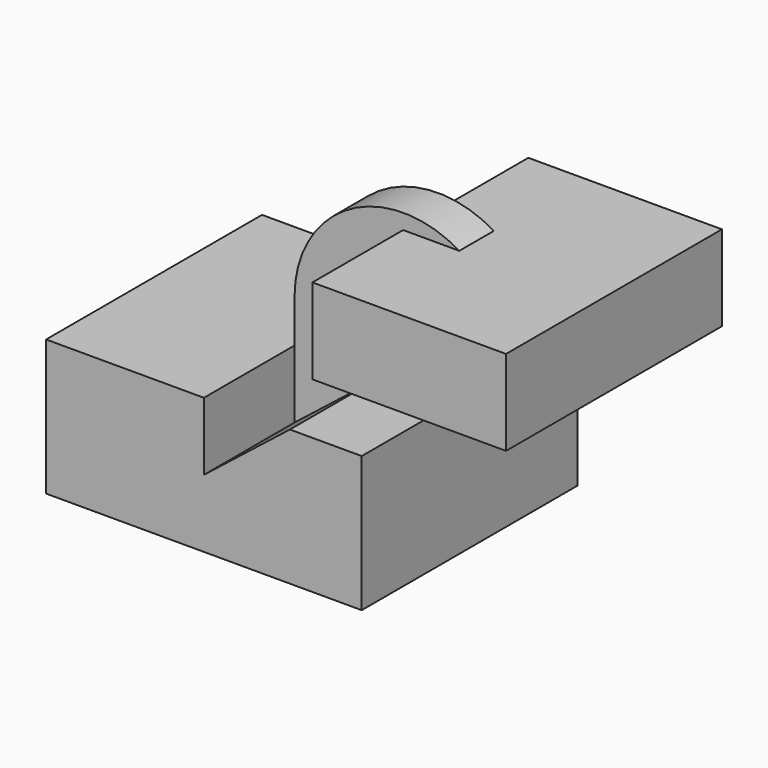
from build123d import *

# Parameters (mm, degrees)
F1_DEPTH = 62.5
F2_DEPTH = 10


with BuildPart() as f1:
    # F0 (on Front) → F1 (new body, symmetric)
    with BuildSketch(Plane.XZ):
        with BuildLine():
            Line((0, 31.4277224243), (-73.1017515063, 31.4277224243))
            Line((-73.1017515063, 31.4277224243), (-73.1017515063, -31.4277224243))
            Line((-73.1017515063, -31.4277224243), (73.1017515063, -31.4277224243))
            Line((73.1017515063, -31.4277224243), (73.1017515063, 31.4277224243))
            Line((73.1017515063, 31.4277224243), (39.8282436226, 31.4277224243))
            add(Edge.make_bspline(
                [(0, 0), (13.2760812075, 10.4759074748), (26.552162415, 20.9518149495), (39.8282436226, 31.4277224243)],
                knots=[0, 0, 0, 0, 50.7345121868, 50.7345121868, 50.7345121868, 50.7345121868], degree=3))
            Line((0, 0), (0, 31.4277224243))
        make_face()
    extrude(amount=F1_DEPTH, both=True)


with BuildPart() as f1b:
    # F0 (on Front) → F1, piece 2 (new body, symmetric)
    with BuildSketch(Plane.XZ):
        with BuildLine():
            add(Edge.make_bspline(
                [(70.0591673961, 55.2823791846), (78.4092683269, 61.8712877179), (86.7593692578, 68.4601962511), (95.1094701886, 75.0491047844)],
                knots=[89.2436461858, 89.2436461858, 89.2436461858, 89.2436461858, 121.1535366735, 121.1535366735, 121.1535366735, 121.1535366735], degree=3))
            Line((70.0591673961, 55.2823791846), (139.946192503, 55.2823791846))
            Line((139.946192503, 55.2823791846), (139.946192503, 94.8158303842))
            Line((139.946192503, 94.8158303842), (76.3028285899, 94.8158303842))
            ThreePointArc((76.3028285899, 94.8158303842), (87.066689677, 86.2269254571), (95.1094701886, 75.0491047844))
        make_face()
        with BuildLine():
            Line((50.2727478743, 55.2823791846), (70.0591673961, 55.2823791846))
            add(Edge.make_bspline(
                [(70.0591673961, 55.2823791846), (78.4092683269, 61.8712877179), (86.7593692578, 68.4601962511), (95.1094701886, 75.0491047844)],
                knots=[89.2436461858, 89.2436461858, 89.2436461858, 89.2436461858, 121.1535366735, 121.1535366735, 121.1535366735, 121.1535366735], degree=3))
            ThreePointArc((95.1094701886, 75.0491047844), (87.066689677, 86.2269254571), (76.3028285899, 94.8158303842))
            Line((76.3028285899, 94.8158303842), (50.2727478743, 94.8158303842))
            Line((50.2727478743, 94.8158303842), (50.2727478743, 55.2823791846))
        make_face()
    extrude(amount=F1_DEPTH, both=True)


with BuildPart() as f2:
    # F0 (on Front) → F2 (new body, symmetric)
    with BuildSketch(Plane.XZ):
        with BuildLine():
            Line((0, 51.4254594788), (0, 31.4277224243))
            Line((0, 31.4277224243), (39.8282436226, 31.4277224243))
            add(Edge.make_bspline(
                [(39.8282436226, 31.4277224243), (49.9052182137, 39.3792746777), (59.9821928049, 47.3308269312), (70.0591673961, 55.2823791846)],
                knots=[50.7345121868, 50.7345121868, 50.7345121868, 50.7345121868, 89.2436461858, 89.2436461858, 89.2436461858, 89.2436461858], degree=3))
            Line((70.0591673961, 55.2823791846), (50.2727478743, 55.2823791846))
            Line((50.2727478743, 55.2823791846), (50.2727478743, 94.8158303842))
            Line((50.2727478743, 94.8158303842), (76.3028285899, 94.8158303842))
            ThreePointArc((76.3028285899, 94.8158303842), (25.5308911631, 95.3140853917), (0, 51.4254594788))
        make_face()
        with BuildLine():
            Line((39.8282436226, 31.4277224243), (0, 31.4277224243))
            Line((0, 31.4277224243), (0, 0))
            add(Edge.make_bspline(
                [(0, 0), (13.2760812075, 10.4759074748), (26.552162415, 20.9518149495), (39.8282436226, 31.4277224243)],
                knots=[0, 0, 0, 0, 50.7345121868, 50.7345121868, 50.7345121868, 50.7345121868], degree=3))
        make_face()
    extrude(amount=F2_DEPTH, both=True)


solid = Compound([f1.part, f1b.part, f2.part])
